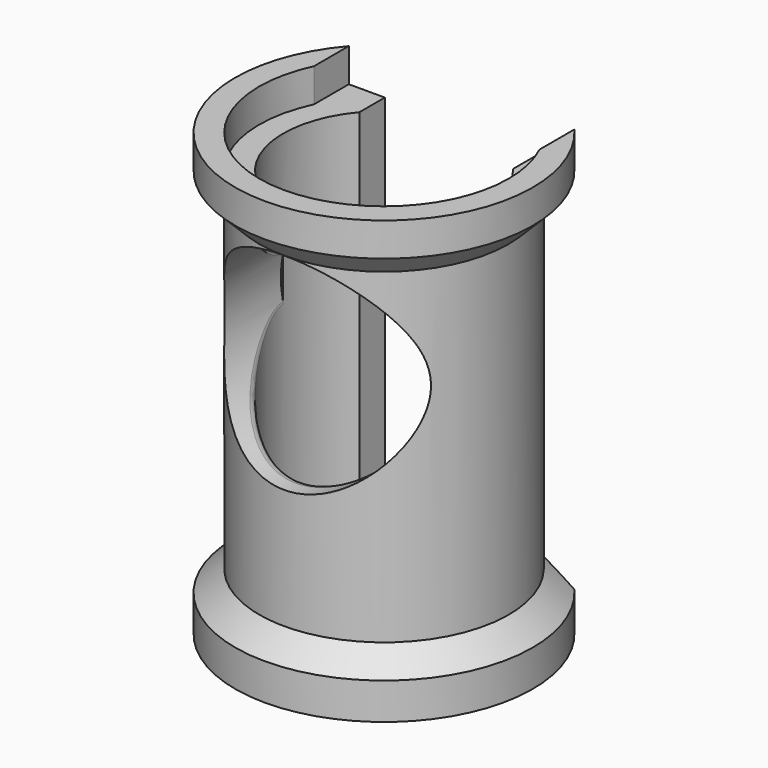
from build123d import *

# Parameters (mm, degrees)
F2_W      = 16
F2_H      = 12.7785220167
F3_DEPTH  = 46.001
F4_W      = 23.5
F4_H      = 13.4564294844
F5_DEPTH  = 3.5
F6_W      = 23.5
F6_H      = 13.0310004231
F7_DEPTH  = 3.8
F8_R      = 10.75
F9_DEPTH  = 25
F11_W     = 31.7701289256
F11_H     = 9.9966360929
F12_DEPTH = 46.001
F14_R     = 1


with BuildPart() as f1:
    # F0 (on Front) → F1 (revolve)
    with BuildSketch(Plane.XZ):
        Polygon((-15.5, 0), (-13, 0), (-13, 3.8), (-10.5, 3.8), (-10.5, 42.5), (-13, 42.5), (-13, 46), (-15.5, 46), (-15.5, 42.5), (-13, 40), (-13, 6), (-15.5, 3.8), align=None)
    revolve(axis=Axis((0, 0, 24.8965322971), (0, 0, 1)))

    # F2 (on face) → F3 (cut, through all)
    with BuildSketch(Plane.XY.offset(46)):
        with Locations((0, 11.7036290467)):
            Rectangle(F2_W, F2_H)
    extrude(amount=-F3_DEPTH, mode=Mode.SUBTRACT)

    # F4 (on face) → F5 (cut, through all)
    with BuildSketch(Plane.XY.offset(46)):
        with Locations((0, 10.8011863194)):
            Rectangle(F4_W, F4_H)
    extrude(amount=-F5_DEPTH, mode=Mode.SUBTRACT)

    # F6 (on face) → F7 (cut, through all)
    with BuildSketch(Plane(origin=(0, 0, 0), x_dir=(1, 0, 0), z_dir=(0, 0, -1))):
        with Locations((0, -9.3560743844)):
            Rectangle(F6_W, F6_H)
    extrude(amount=-F7_DEPTH, mode=Mode.SUBTRACT)

    # F8 (on Front) → F9 (cut)
    with BuildSketch(Plane.XZ):
        with Locations((0, 29.25)):
            Circle(F8_R)
    extrude(amount=F9_DEPTH, mode=Mode.SUBTRACT)

    # F11 (on Top) → F12 (cut, through all)
    with BuildSketch(Plane.XY):
        with Locations((0.0608135015, 15.107101356)):
            Rectangle(F11_W, F11_H)
    extrude(amount=F12_DEPTH, mode=Mode.SUBTRACT)

    # F14
    f14_edges = [f1.edges().sort_by_distance(p)[0] for p in [
        (0.039521, -10.499926, 18.500073),
    ]]
    fillet(f14_edges, radius=F14_R)


solid = f1.part
